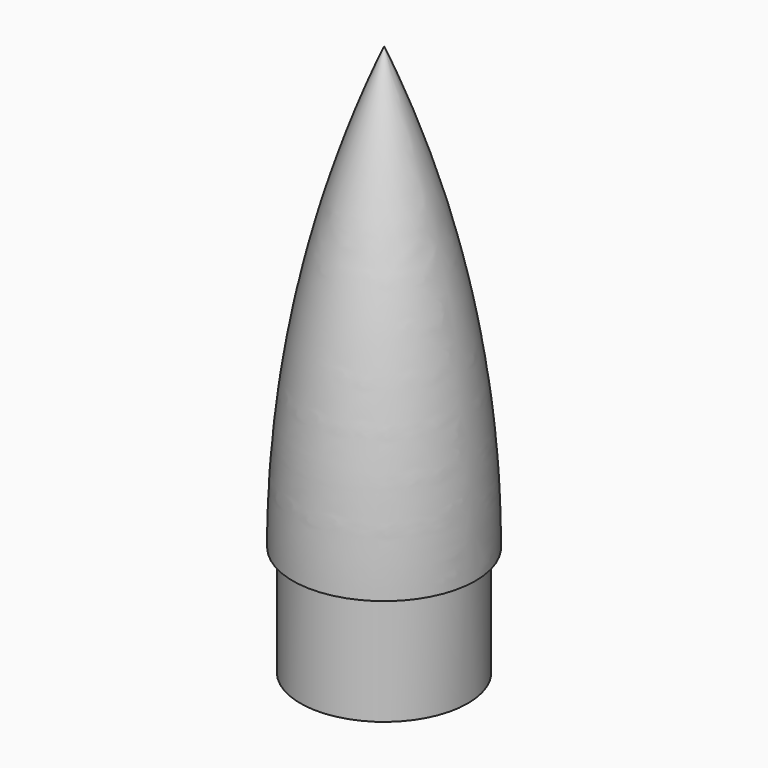
from build123d import *


# Not quite as in the source:
# - a fillet or chamfer that OpenCascade refuses, or shapes differently, is made with other operations: its cross-section is extruded or revolved along the edge and cut away or added


with BuildPart() as f1:
    # F0 (on Front) → F1 (revolve)
    with BuildSketch(Plane.XZ):
        with BuildLine():
            Line((16.3, 28.4), (16.3, 0))
            Line((16.3, 0), (19.3, 0))
            Line((19.3, 0), (19.3, 25.4))
            Line((19.3, 25.4), (21.05, 25.4))
            ThreePointArc((21.05, 25.4), (15.7322064745, 77.2788552784), (0, 127))
            Line((0, 127), (0, 119.1937167747))
            ThreePointArc((0, 119.1937167747), (13.2086358673, 74.6295226115), (18.0321928546, 28.4))
            Line((18.0321928546, 28.4), (16.3, 28.4))
        make_face()
    revolve(axis=Axis((0, 0, 63.5), (0, 0, 1)))

    # F2: fillet of radius 5.08 on 1 edges, made by hand

    # F2_s1 → F2_t2 (revolve)
    with BuildSketch(Plane.XZ):
        with BuildLine():
            ThreePointArc((17.9559785466, 32.2929453531), (17.5525109987, 30.1658899028), (16.3, 28.4))
            Line((16.3, 28.4), (18.0321928546, 28.4))
            ThreePointArc((18.0321928546, 28.4), (18.0015833093, 30.3466194613), (17.9559785466, 32.2929453531))
        make_face()
    revolve(axis=Axis((0, 0, 28.4), (0, 0, 1)))


solid = f1.part
